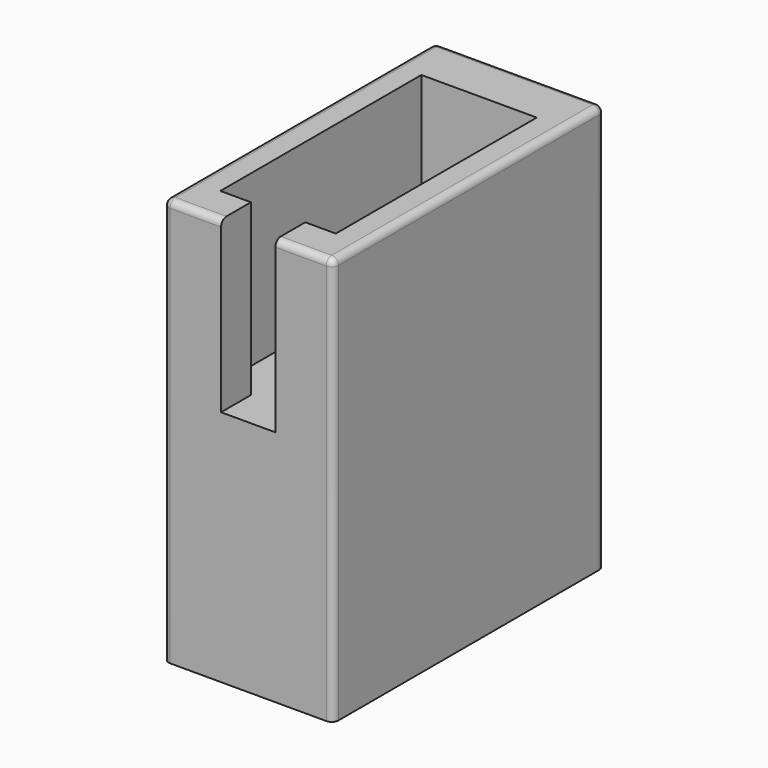
from build123d import *

# Parameters (mm, degrees)
F0_W         = 25
F0_H         = 50
F1_DEPTH     = 60
F2_R         = 1
F4_DEPTH     = 25
F5_T1_DEPTH  = 10
F5_T3_DEPTH  = 10
F5_S7_W      = 1
F5_S7_H      = 1
F5_T8_DEPTH  = 1
F5_S13_W     = 1
F5_S13_H     = 1
F5_T14_DEPTH = 1


# Not quite as in the source:
# - a fillet or chamfer that OpenCascade refuses, or shapes differently, is made with other operations: its cross-section is extruded or revolved along the edge and cut away or added


with BuildPart() as f1:
    # F0 (on Top) → F1 (new body)
    with BuildSketch(Plane.XY):
        with Locations((12.5, 25)):
            Rectangle(F0_W, F0_H)
    extrude(amount=F1_DEPTH)

    # F2
    f2_edges = [f1.edges().sort_by_distance(p)[0] for p in [
        (0, 25, 60),
        (12.5, 50, 60),
        (25, 25, 60),
        (25, 0, 30),
        (0, 0, 30),
        (0, 50, 30),
        (25, 50, 30),
    ]]
    fillet(f2_edges, radius=F2_R)

    # F3 (on face) → F4 (cut)
    with BuildSketch(Plane.XY.offset(60)):
        Polygon((21, 42.5), (4, 42.5), (4, 5.5), (8.5, 5.5), (8.5, 0), (16.5, 0), (16.5, 5.5), (21, 5.5), align=None)
    extrude(amount=-F4_DEPTH, mode=Mode.SUBTRACT)

    # F5: fillet of radius 1 on 2 edges, made by hand

    # F5_s2 → F5_t1 (cut)
    with BuildSketch(Plane.YZ.offset(1)):
        with BuildLine():
            ThreePointArc((0, 59), (0.2928932188, 59.7071067812), (1, 60))
            Line((1, 60), (0, 60))
            Line((0, 60), (0, 59))
        make_face()
    extrude(amount=F5_T1_DEPTH, mode=Mode.SUBTRACT)

    # F5_s4 → F5_t3 (cut)
    with BuildSketch(Plane.YZ.offset(14)):
        with BuildLine():
            ThreePointArc((0, 59), (0.2928932188, 59.7071067812), (1, 60))
            Line((1, 60), (0, 60))
            Line((0, 60), (0, 59))
        make_face()
    extrude(amount=F5_T3_DEPTH, mode=Mode.SUBTRACT)


with BuildPart() as f5_tool6:
    # F5_s7 → F5_t8 (new body)
    with BuildSketch(Plane.XZ.offset(-1)):
        with Locations((24.5, 59.5)):
            Rectangle(F5_S7_W, F5_S7_H)
    extrude(amount=F5_T8_DEPTH)

    # F5_s9 → F5_t10 (revolve, cut)
    with BuildSketch(Plane(origin=(24, 1, 59), x_dir=(-0.7071067812, 0, -0.7071067812), z_dir=(-0.7071067812, 0, 0.7071067812))):
        with BuildLine():
            ThreePointArc((0, -1), (1, 0), (0, 1))
            Line((0, 1), (0, -1))
        make_face()
    revolve(axis=Axis((24, 1, 59), (0, -1, 0)), mode=Mode.SUBTRACT)


with BuildPart() as f1_1:
    add(f1.part)

    # F5_t5: cut F5_tool6
    add(f5_tool6.part, mode=Mode.SUBTRACT)


with BuildPart() as f5_tool12:
    # F5_s13 → F5_t14 (new body)
    with BuildSketch(Plane.XZ.offset(-1)):
        with Locations((0.5, 59.5)):
            Rectangle(F5_S13_W, F5_S13_H)
    extrude(amount=F5_T14_DEPTH)

    # F5_s15 → F5_t16 (revolve, cut)
    with BuildSketch(Plane(origin=(1, 1, 59), x_dir=(0.7071067812, 0, -0.7071067812), z_dir=(-0.7071067812, 0, -0.7071067812))):
        with BuildLine():
            ThreePointArc((0, -1), (1, 0), (0, 1))
            Line((0, 1), (0, -1))
        make_face()
    revolve(axis=Axis((1, 1, 59), (0, -1, 0)), mode=Mode.SUBTRACT)


with BuildPart() as f1_2:
    add(f1_1.part)

    # F5_t11: cut F5_tool12
    add(f5_tool12.part, mode=Mode.SUBTRACT)


solid = f1_2.part
